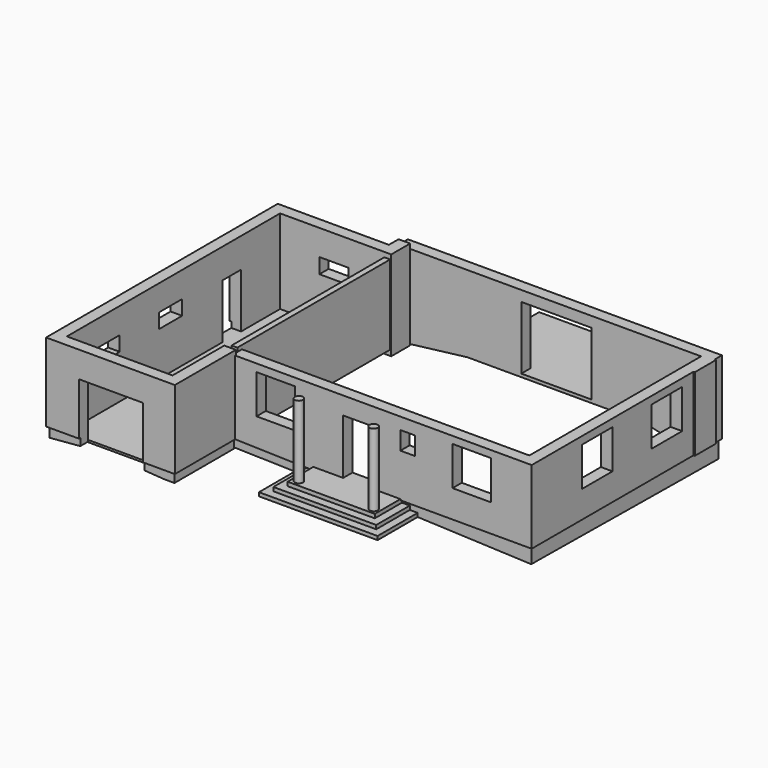
from build123d import *

# Parameters (mm, degrees)
F1_DEPTH      = 440
F2_DEPTH      = 370
F3_W          = 1110
F3_H          = 560
F4_DEPTH      = 370
F4_DEPTH_BACK = 70
F5_DEPTH      = 370
F6_W          = 3785
F6_H          = 2980
F6_W_2        = 1105
F6_H_2        = 575
F7_DEPTH      = 440
F6_W_3        = 370
F6_H_3        = 410
F8_DEPTH      = 370
F9_DEPTH      = 900
F6_H_4        = 430
F10_DEPTH     = 900
F11_W         = 190
F11_H         = 1765
F12_DEPTH     = 400
F14_DEPTH     = 440
F15_DEPTH     = 370
F16_DEPTH     = 3415
F18_DEPTH     = 440
F17_W         = 7250
F17_H         = 2800
F17_W_2       = 1460
F17_H_2       = 1480
F17_W_3       = 910
F17_W_4       = 100
F19_DEPTH     = 490
F20_DEPTH     = 370
F21_W         = 1460
F21_H         = 1480
F21_W_2       = 1470
F21_W_3       = 550
F21_H_2       = 690
F22_DEPTH     = 440
F23_DEPTH     = 370
F24_DEPTH     = 2275
F25_DEPTH     = 1965
F26_DEPTH     = 1660
F27_R         = 155
F28_DEPTH     = 2765
F29_W         = 2460
F29_H         = 2980
F30_DEPTH     = 440
F29_H_2       = 350
F29_W_2       = 370
F31_DEPTH     = 370
F33_DEPTH     = 80
F34_W         = 220
F34_H         = 900
F34_H_2       = 7260
F35_DEPTH     = 3020


with BuildPart() as f1:
    # F0 (on Front) → F1 (new body)
    with BuildSketch(Plane.XZ):
        Polygon((0, 2980), (0, 0), (70, 0), (1245, 0), (1245, 1990), (3685, 1990), (3685, 0), (4455, 0), (4455, 2980), align=None)
    extrude(amount=F1_DEPTH)

    # F0 (on Front) → F2 (join)
    with BuildSketch(Plane.XZ):
        Polygon((1245, 0), (70, 0), (70, -380), (1245, -280), (1245, -180), align=None)
        Polygon((4455, -350), (4455, 0), (3685, 0), (3685, -180), (3685, -300), align=None)
    extrude(amount=F2_DEPTH)

    # F3 (on face) → F4 (join, two sides)
    with BuildSketch(Plane(origin=(70, 0, 0), x_dir=(0, -1, 0), z_dir=(-1, 0, 0))) as f4_sk:
        Polygon((440, 0), (440, 2980), (-10130, 2980), (-10130, 0), (-8275, 0), (-8275, 1850), (-7385, 1850), (-7385, 0), (0, 0), (370, 0), align=None)
        with Locations((-4920, 1725)):
            Rectangle(F3_W, F3_H, mode=Mode.SUBTRACT)
        with Locations((-1955, 1725)):
            Rectangle(F3_W, F3_H, mode=Mode.SUBTRACT)
    extrude(amount=-F4_DEPTH)
    extrude(f4_sk.sketch, amount=F4_DEPTH_BACK)

    # F3 (on face) → F5 (join)
    with BuildSketch(Plane(origin=(70, 0, 0), x_dir=(0, -1, 0), z_dir=(-1, 0, 0))):
        Polygon((-8275, 0), (-10130, 0), (-10130, -410), (0, -380), (0, 0), (-7385, 0), (-7385, -220), (-8275, -220), align=None)
    extrude(amount=-F5_DEPTH)

    # F6 (on face) → F7 (join)
    with BuildSketch(Plane(origin=(0, 10130, 0), x_dir=(-1, 0, 0), z_dir=(0, 1, 0))):
        Polygon((0, 0), (0, 2980), (-440, 2980), (-440, 0), (-70, 0), align=None)
        with Locations((-2332.5, 1490)):
            Rectangle(F6_W, F6_H)
        with Locations((-2487.5, 1717.5)):
            Rectangle(F6_W_2, F6_H_2, mode=Mode.SUBTRACT)
    extrude(amount=F7_DEPTH)

    # F6 (on face) → F8 (join)
    with BuildSketch(Plane(origin=(0, 10130, 0), x_dir=(-1, 0, 0), z_dir=(0, 1, 0))):
        Polygon((-440, -410), (-440, 0), (-4225, 0), (-4295, 0), (-4295, -430), (-70, -410), align=None)
        with Locations((-255, -205)):
            Rectangle(F6_W_3, F6_H_3)
    extrude(amount=F8_DEPTH)

    # F6 (on face) → F9 (join)
    with BuildSketch(Plane(origin=(0, 10130, 0), x_dir=(-1, 0, 0), z_dir=(0, 1, 0))):
        Polygon((-4225, 0), (-4225, 2980), (-4665, 2980), (-4665, 0), (-4295, 0), align=None)
    extrude(amount=F9_DEPTH)

    # F6 (on face) → F10 (join)
    with BuildSketch(Plane(origin=(0, 10130, 0), x_dir=(-1, 0, 0), z_dir=(0, 1, 0))):
        with Locations((-4480, -215)):
            Rectangle(F6_W_3, F6_H_4)
    extrude(amount=F10_DEPTH)

    # F11 (on face) → F12 (cut)
    with BuildSketch(Plane(origin=(4225, 0, 0), x_dir=(0, -1, 0), z_dir=(-1, 0, 0))):
        with Locations((-10785, 1402.5)):
            Rectangle(F11_W, F11_H)
    extrude(amount=-F12_DEPTH, mode=Mode.SUBTRACT)

    # F13 (on face) → F14 (join)
    with BuildSketch(Plane(origin=(0, 11030, 0), x_dir=(-1, 0, 0), z_dir=(0, 1, 0))):
        Polygon((-6835, 0), (-4665, 0), (-4665, 2800), (-15725, 2800), (-15725, 0), (-13595, 0), (-11550, 0), (-11550, 2400), (-8890, 2400), (-8890, 0), align=None)
        Polygon((-4295, 0), (-4225, 0), (-4225, 2800), (-4665, 2800), (-4665, 0), align=None)
    extrude(amount=F14_DEPTH)

    # F13 (on face) → F15 (join)
    with BuildSketch(Plane(origin=(0, 11030, 0), x_dir=(-1, 0, 0), z_dir=(0, 1, 0))):
        Polygon((-13595, 0), (-15725, 0), (-15725, -660), (-13595, -120), align=None)
        Polygon((-4665, -384.842519685), (-4665, 0), (-6835, 0), (-6835, -120), align=None)
        Polygon((-4295, -430), (-4295, 0), (-4665, 0), (-4665, -384.842519685), align=None)
    extrude(amount=F15_DEPTH)

    # F13 (on face) → F16 (join)
    with BuildSketch(Plane(origin=(0, 11030, 0), x_dir=(-1, 0, 0), z_dir=(0, 1, 0))):
        Polygon((-6835, -120), (-6835, 0), (-8890, 0), (-11550, 0), (-13595, 0), (-13595, -120), align=None)
    extrude(amount=F16_DEPTH)

    # F17 (on face) → F18 (join)
    with BuildSketch(Plane.YZ.offset(15725)):
        Polygon((11400, 0), (11470, 0), (11470, 2800), (11130, 2800), (11130, 0), align=None)
    extrude(amount=F18_DEPTH)



with BuildPart() as f18:
    # F17 (on face) → F18, piece 2 (new body)
    with BuildSketch(Plane.YZ.offset(15725)):
        with Locations((6495, 1400)):
            Rectangle(F17_W, F17_H)
        with Locations((5540, 1770)):
            Rectangle(F17_W_2, F17_H_2, mode=Mode.SUBTRACT)
        with Locations((8850, 1770)):
            Rectangle(F17_W_2, F17_H_2, mode=Mode.SUBTRACT)
    extrude(amount=F18_DEPTH)


with BuildPart() as f1_1:
    add(f1.part)

    add(f18.part)  # F19 merges F18
    # F17 (on face) → F19 (join)
    with BuildSketch(Plane.YZ.offset(15725)):
        with Locations((10575, 1400)):
            Rectangle(F17_W_3, F17_H)
        with Locations((11080, 1400)):
            Rectangle(F17_W_4, F17_H)
    extrude(amount=F19_DEPTH)

    # F17 (on face) → F20 (join)
    with BuildSketch(Plane.YZ.offset(15725)):
        Polygon((11030, -656.0961313013), (11030, 0), (10120, 0), (2870, 0), (2870, -570), align=None)
        Polygon((11400, -660), (11400, 0), (11130, 0), (11030, 0), (11030, -656.0961313013), align=None)
    extrude(amount=F20_DEPTH)

    # F21 (on face) → F22 (join)
    with BuildSketch(Plane.XZ.offset(-2870)):
        Polygon((15725, 0), (15725, 2800), (4800, 2800), (4800, 0), (7865, -79.944847658), (7865, 40.055152342), (9000, 40.055152342), (9000, 2130.055152342), (10040, 2130.055152342), (10040, 40.055152342), (11175, 40.055152342), (11175, 0), align=None)
        with Locations((6435, 1770)):
            Rectangle(F21_W, F21_H, mode=Mode.SUBTRACT)
        with Locations((13890, 1790)):
            Rectangle(F21_W_2, F21_H, mode=Mode.SUBTRACT)
        with Locations((11450, 2005)):
            Rectangle(F21_W_3, F21_H_2, mode=Mode.SUBTRACT)
        Polygon((16165, 0), (16165, 2800), (15725, 2800), (15725, 0), (16095, 0), align=None)
    extrude(amount=F22_DEPTH)

    # F21 (on face) → F23 (join)
    with BuildSketch(Plane.XZ.offset(-2870)):
        Polygon((15725, -555.0068503781), (15725, 0), (11175, 0), (11175, -109.944847658), (11475, -109.944847658), (11475, -254.944847658), (11775, -254.944847658), (11775, -394.944847658), align=None)
        Polygon((16095, 0), (15725, 0), (15725, -555.0068503781), (16095, -570), align=None)
        Polygon((7865, -79.944847658), (4800, 0), (4730, 0), (4730, -330), (7265, -394.944847658), (7265, -254.944847658), (7565, -254.944847658), (7565, -109.944847658), (7865, -109.944847658), align=None)
    extrude(amount=F23_DEPTH)

    # F21 (on face) → F24 (join)
    with BuildSketch(Plane.XZ.offset(-2870)):
        Polygon((7265, -394.944847658), (11775, -394.944847658), (11775, -254.944847658), (11475, -254.944847658), (7565, -254.944847658), (7265, -254.944847658), align=None)
    extrude(amount=F24_DEPTH)

    # F21 (on face) → F25 (join)
    with BuildSketch(Plane.XZ.offset(-2870)):
        Polygon((11475, -109.944847658), (11175, -109.944847658), (7865, -109.944847658), (7565, -109.944847658), (7565, -254.944847658), (11475, -254.944847658), align=None)
    extrude(amount=F25_DEPTH)

    # F21 (on face) → F26 (join)
    with BuildSketch(Plane.XZ.offset(-2870)):
        Polygon((11175, -109.944847658), (11175, 0), (11175, 40.055152342), (10040, 40.055152342), (9000, 40.055152342), (7865, 40.055152342), (7865, -79.944847658), (7865, -109.944847658), align=None)
    extrude(amount=F26_DEPTH)

    # F27 (on face) → F28 (join)
    with BuildSketch(Plane.XY.offset(40.055152342)):
        with Locations((8095, 1455)):
            Circle(F27_R)
        with Locations((10950, 1440)):
            Circle(F27_R)
    extrude(amount=F28_DEPTH)

    # F29 (on face) → F30 (join)
    with BuildSketch(Plane.YZ.offset(4455)):
        with Locations((1230, 1490)):
            Rectangle(F29_W, F29_H)
        Polygon((0, 0), (0, 2980), (-440, 2980), (-440, 0), (-370, 0), align=None)
    extrude(amount=F30_DEPTH)

    # F29 (on face) → F31 (join)
    with BuildSketch(Plane.YZ.offset(4455)):
        with Locations((1230, -175)):
            Rectangle(F29_W, F29_H_2)
        with Locations((-185, -175)):
            Rectangle(F29_W_2, F29_H_2)
    extrude(amount=F31_DEPTH)

    # F32 (on face) → F33 (join)
    with BuildSketch(Plane.XY.offset(-220)):
        Polygon((440, 10130), (440, 8275), (440, 7385), (440, 0), (4455, 0), (4440, 10130), align=None)
    extrude(amount=-F33_DEPTH)

    # F34 (on face) → F35 (join)
    with BuildSketch(Plane.XY.offset(2800)):
        with Locations((4515, 10580)):
            Rectangle(F34_W, F34_H)
        with Locations((4515, 6500)):
            Rectangle(F34_W, F34_H_2)
    extrude(amount=-F35_DEPTH)


solid = f1_1.part
